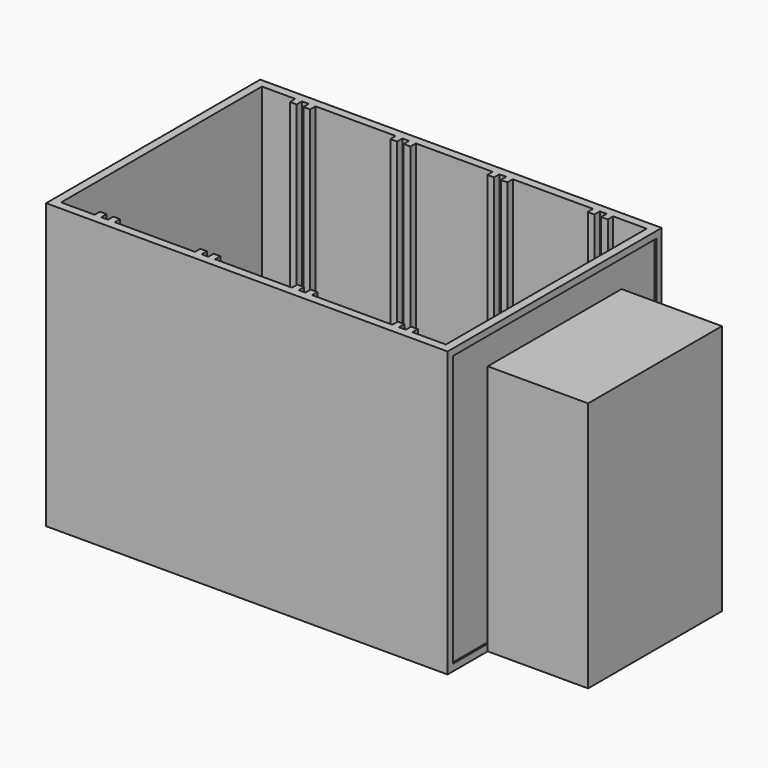
from build123d import *

# Parameters (mm, degrees)
F0_W           = 120
F0_H           = 80
F1_DEPTH       = 85
F2_T           = -2.5
F3_W           = 2
F3_H           = 2
F4_DEPTH       = 85
F5_W           = 30
F5_H           = 50
F6_DEPTH       = 75
F7_T           = -2
F7_2_T         = 2
F7_2_T3_DEPTH  = 86.5
F7_2_T5_DEPTH  = 14
F7_2_T7_DEPTH  = 6
F7_2_T9_DEPTH  = 28
F7_2_T11_DEPTH = 6
F7_2_T13_DEPTH = 27
F7_2_T15_DEPTH = 6
F7_2_T17_DEPTH = 28
F7_2_T19_DEPTH = 6
F7_2_T21_DEPTH = 14
F7_2_T23_DEPTH = 79
F7_2_T25_DEPTH = 6
F7_2_T27_DEPTH = 6
F7_2_T29_DEPTH = 6
F7_2_T31_DEPTH = 6
F7_2_T33_DEPTH = 6
F7_2_T35_DEPTH = 6
F7_2_T37_DEPTH = 6
F7_2_T39_DEPTH = 6
F7_2_T41_DEPTH = 6
F7_2_T43_DEPTH = 6


# Not quite as in the source:
# - a shell that OpenCascade refuses in one call is made with other operations: the cavity is built on its own and cut out


with BuildPart() as f1:
    # F0 (on Top) → F1 (new body)
    with BuildSketch(Plane.XY):
        Rectangle(F0_W, F0_H)
    extrude(amount=F1_DEPTH)

    # F2
    f2_openings = [f1.faces().sort_by_distance(p)[0] for p in [
        (0, 0, 85),
    ]]
    offset(amount=F2_T, openings=f2_openings)

    # F3 (on Top) → F4 (join)
    with BuildSketch(Plane.XY):
        with Locations((-46.5, -36.5)):
            Rectangle(F3_W, F3_H)
        with Locations((-42.5, -36.5)):
            Rectangle(F3_W, F3_H)
        with Locations((-16.5, -36.5)):
            Rectangle(F3_W, F3_H)
        with Locations((-12.5, -36.5)):
            Rectangle(F3_W, F3_H)
        with Locations((42.5, -36.5)):
            Rectangle(F3_W, F3_H)
        with Locations((46.5, -36.5)):
            Rectangle(F3_W, F3_H)
        with Locations((12.5, -36.5)):
            Rectangle(F3_W, F3_H)
        with Locations((16.5, -36.5)):
            Rectangle(F3_W, F3_H)
        with Locations((-46.5, 36.5)):
            Rectangle(F3_W, F3_H)
        with Locations((42.5, 36.5)):
            Rectangle(F3_W, F3_H)
        with Locations((-16.5, 36.5)):
            Rectangle(F3_W, F3_H)
        with Locations((-42.5, 36.5)):
            Rectangle(F3_W, F3_H)
        with Locations((-12.5, 36.5)):
            Rectangle(F3_W, F3_H)
        with Locations((46.5, 36.5)):
            Rectangle(F3_W, F3_H)
        with Locations((16.5, 36.5)):
            Rectangle(F3_W, F3_H)
        with Locations((12.5, 36.5)):
            Rectangle(F3_W, F3_H)
    extrude(amount=F4_DEPTH)

    # F7#2: shell of thickness 2, made by hand


with BuildPart() as f6:
    # F5 (on Top) → F6 (new body)
    with BuildSketch(Plane.XY):
        with Locations((75, 0)):
            Rectangle(F5_W, F5_H)
    extrude(amount=F6_DEPTH)

    # F7
    f7_openings = [f6.faces().sort_by_distance(p)[0] for p in [
        (60, 0, 37.5),
    ]]
    offset(amount=F7_T, openings=f7_openings)


with BuildPart() as f7_2_core1:
    # F7_2_t2: copy of F1
    add(f1.part)

    # the walls: a layer under each face that stays
    f7_2_faces = [f7_2_core1.faces().sort_by_distance(p)[0] for p in [
        (0, -40, 42.5),
        (-60, 0, 42.5),
        (0, 0, 0),
        (-16, -37.3333333333, 85),
        (0, 40, 42.5),
        (-52.5, -37.5, 43.75),
        (-44.5, -37.5, 43.75),
        (-29.5, -37.5, 43.75),
        (-14.5, -37.5, 43.75),
        (0, -37.5, 43.75),
        (14.5, -37.5, 43.75),
        (29.5, -37.5, 43.75),
        (44.5, -37.5, 43.75),
        (52.5, -37.5, 43.75),
        (-57.5, 0, 43.75),
        (52.5, 37.5, 43.75),
        (44.5, 37.5, 43.75),
        (29.5, 37.5, 43.75),
        (14.5, 37.5, 43.75),
        (0, 37.5, 43.75),
        (-14.5, 37.5, 43.75),
        (-29.5, 37.5, 43.75),
        (-44.5, 37.5, 43.75),
        (-52.5, 37.5, 43.75),
        (57.5, 0, 43.75),
        (0, 0, 2.5),
        (-47.5, -36.5, 43.75),
        (-45.5, -36.5, 43.75),
        (-46.5, -35.5, 43.75),
        (-43.5, -36.5, 43.75),
        (-41.5, -36.5, 43.75),
        (-42.5, -35.5, 43.75),
        (-17.5, -36.5, 43.75),
        (-15.5, -36.5, 43.75),
        (-16.5, -35.5, 43.75),
        (-13.5, -36.5, 43.75),
        (-11.5, -36.5, 43.75),
        (-12.5, -35.5, 43.75),
        (11.5, -36.5, 43.75),
        (12.5, -35.5, 43.75),
        (13.5, -36.5, 43.75),
        (15.5, -36.5, 43.75),
        (17.5, -36.5, 43.75),
        (16.5, -35.5, 43.75),
        (41.5, -36.5, 43.75),
        (43.5, -36.5, 43.75),
        (42.5, -35.5, 43.75),
        (45.5, -36.5, 43.75),
        (47.5, -36.5, 43.75),
        (46.5, -35.5, 43.75),
        (47.5, 36.5, 43.75),
        (46.5, 35.5, 43.75),
        (45.5, 36.5, 43.75),
        (43.5, 36.5, 43.75),
        (42.5, 35.5, 43.75),
        (41.5, 36.5, 43.75),
        (17.5, 36.5, 43.75),
        (15.5, 36.5, 43.75),
        (16.5, 35.5, 43.75),
        (13.5, 36.5, 43.75),
        (11.5, 36.5, 43.75),
        (12.5, 35.5, 43.75),
        (-11.5, 36.5, 43.75),
        (-13.5, 36.5, 43.75),
        (-12.5, 35.5, 43.75),
        (-15.5, 36.5, 43.75),
        (-17.5, 36.5, 43.75),
        (-16.5, 35.5, 43.75),
        (-41.5, 36.5, 43.75),
        (-43.5, 36.5, 43.75),
        (-42.5, 35.5, 43.75),
        (-45.5, 36.5, 43.75),
        (-46.5, 35.5, 43.75),
        (-47.5, 36.5, 43.75),
    ]]
    thicken(f7_2_faces, amount=-F7_2_T, mode=Mode.SUBTRACT)

    # F7_2_s4 → F7_2_t3 (cut)
    with BuildSketch(Plane.XY.offset(0.5)):
        Polygon((-57.48, -37.48), (-57.5, -39.5), (-59.5, -39.5), (-59.5, -37.5), align=None)
        Polygon((-47.52, -37.48), (-47.5, -39.5), (-45.5, -39.5), (-45.5, -37.5), align=None)
        Polygon((-45.48, -37.48), (-45.5, -39.5), (-47.5, -39.5), (-47.5, -37.5), align=None)
        Polygon((-43.52, -37.48), (-43.5, -39.5), (-41.5, -39.5), (-41.5, -37.5), align=None)
        Polygon((-41.48, -37.48), (-41.5, -39.5), (-43.5, -39.5), (-43.5, -37.5), align=None)
        Polygon((-17.52, -37.48), (-17.5, -39.5), (-15.5, -39.5), (-15.5, -37.5), align=None)
        Polygon((-15.48, -37.48), (-15.5, -39.5), (-17.5, -39.5), (-17.5, -37.5), align=None)
        Polygon((-13.52, -37.48), (-13.5, -39.5), (-11.5, -39.5), (-11.5, -37.5), align=None)
        Polygon((-11.48, -37.48), (-11.5, -39.5), (-13.5, -39.5), (-13.5, -37.5), align=None)
        Polygon((11.48, -37.48), (11.5, -39.5), (13.5, -39.5), (13.5, -37.5), align=None)
        Polygon((13.52, -37.48), (13.5, -39.5), (11.5, -39.5), (11.5, -37.5), align=None)
        Polygon((15.48, -37.48), (15.5, -39.5), (17.5, -39.5), (17.5, -37.5), align=None)
        Polygon((17.52, -37.48), (17.5, -39.5), (15.5, -39.5), (15.5, -37.5), align=None)
        Polygon((41.48, -37.48), (41.5, -39.5), (43.5, -39.5), (43.5, -37.5), align=None)
        Polygon((43.52, -37.48), (43.5, -39.5), (41.5, -39.5), (41.5, -37.5), align=None)
        Polygon((45.48, -37.48), (45.5, -39.5), (47.5, -39.5), (47.5, -37.5), align=None)
        Polygon((47.52, -37.48), (47.5, -39.5), (45.5, -39.5), (45.5, -37.5), align=None)
        Polygon((57.48, -37.48), (57.5, -39.5), (59.5, -39.5), (59.5, -37.5), align=None)
        Polygon((-57.48, 37.48), (-59.5, 37.5), (-59.5, 39.5), (-57.5, 39.5), align=None)
        Polygon((57.48, 37.48), (57.5, 39.5), (59.5, 39.5), (59.5, 37.5), align=None)
        Polygon((47.52, 37.48), (47.5, 39.5), (45.5, 39.5), (45.5, 37.5), align=None)
        Polygon((45.48, 37.48), (45.5, 39.5), (47.5, 39.5), (47.5, 37.5), align=None)
        Polygon((43.52, 37.48), (43.5, 39.5), (41.5, 39.5), (41.5, 37.5), align=None)
        Polygon((41.48, 37.48), (41.5, 39.5), (43.5, 39.5), (43.5, 37.5), align=None)
        Polygon((17.52, 37.48), (17.5, 39.5), (15.5, 39.5), (15.5, 37.5), align=None)
        Polygon((15.48, 37.48), (15.5, 39.5), (17.5, 39.5), (17.5, 37.5), align=None)
        Polygon((13.52, 37.48), (13.5, 39.5), (11.5, 39.5), (11.5, 37.5), align=None)
        Polygon((11.48, 37.48), (11.5, 39.5), (13.5, 39.5), (13.5, 37.5), align=None)
        Polygon((-11.48, 37.48), (-11.5, 39.5), (-13.5, 39.5), (-13.5, 37.5), align=None)
        Polygon((-13.52, 37.48), (-13.5, 39.5), (-11.5, 39.5), (-11.5, 37.5), align=None)
        Polygon((-15.48, 37.48), (-15.5, 39.5), (-17.5, 39.5), (-17.5, 37.5), align=None)
        Polygon((-17.52, 37.48), (-17.5, 39.5), (-15.5, 39.5), (-15.5, 37.5), align=None)
        Polygon((-41.48, 37.48), (-41.5, 39.5), (-43.5, 39.5), (-43.5, 37.5), align=None)
        Polygon((-43.52, 37.48), (-43.5, 39.5), (-41.5, 39.5), (-41.5, 37.5), align=None)
        Polygon((-45.48, 37.48), (-45.5, 39.5), (-47.5, 39.5), (-47.5, 37.5), align=None)
        Polygon((-47.52, 37.48), (-47.5, 39.5), (-45.5, 39.5), (-45.5, 37.5), align=None)
    extrude(amount=F7_2_T3_DEPTH, mode=Mode.SUBTRACT)

    # F7_2_s6 → F7_2_t5 (cut)
    with BuildSketch(Plane.YZ.offset(-59.5)):
        Polygon((-37.48, 2.52), (-39.5, 2.5), (-39.5, 0.5), (-37.5, 0.5), align=None)
        Polygon((37.48, 2.52), (39.5, 2.5), (39.5, 0.5), (37.5, 0.5), align=None)
    extrude(amount=F7_2_T5_DEPTH, mode=Mode.SUBTRACT)

    # F7_2_s8 → F7_2_t7 (cut)
    with BuildSketch(Plane.YZ.offset(-47.5)):
        Polygon((-37.48, 2.52), (-39.5, 2.5), (-39.5, 0.5), (-37.5, 0.5), align=None)
        Polygon((37.48, 2.52), (39.5, 2.5), (39.5, 0.5), (37.5, 0.5), align=None)
    extrude(amount=F7_2_T7_DEPTH, mode=Mode.SUBTRACT)

    # F7_2_s10 → F7_2_t9 (cut)
    with BuildSketch(Plane.YZ.offset(-43.5)):
        Polygon((-37.48, 2.52), (-39.5, 2.5), (-39.5, 0.5), (-37.5, 0.5), align=None)
        Polygon((37.48, 2.52), (39.5, 2.5), (39.5, 0.5), (37.5, 0.5), align=None)
    extrude(amount=F7_2_T9_DEPTH, mode=Mode.SUBTRACT)

    # F7_2_s12 → F7_2_t11 (cut)
    with BuildSketch(Plane.YZ.offset(-17.5)):
        Polygon((-37.48, 2.52), (-39.5, 2.5), (-39.5, 0.5), (-37.5, 0.5), align=None)
        Polygon((37.48, 2.52), (39.5, 2.5), (39.5, 0.5), (37.5, 0.5), align=None)
    extrude(amount=F7_2_T11_DEPTH, mode=Mode.SUBTRACT)

    # F7_2_s14 → F7_2_t13 (cut)
    with BuildSketch(Plane.YZ.offset(-13.5)):
        Polygon((-37.48, 2.52), (-39.5, 2.5), (-39.5, 0.5), (-37.5, 0.5), align=None)
        Polygon((37.48, 2.52), (39.5, 2.5), (39.5, 0.5), (37.5, 0.5), align=None)
    extrude(amount=F7_2_T13_DEPTH, mode=Mode.SUBTRACT)

    # F7_2_s16 → F7_2_t15 (cut)
    with BuildSketch(Plane.YZ.offset(11.5)):
        Polygon((-37.48, 2.52), (-39.5, 2.5), (-39.5, 0.5), (-37.5, 0.5), align=None)
        Polygon((37.48, 2.52), (39.5, 2.5), (39.5, 0.5), (37.5, 0.5), align=None)
    extrude(amount=F7_2_T15_DEPTH, mode=Mode.SUBTRACT)

    # F7_2_s18 → F7_2_t17 (cut)
    with BuildSketch(Plane.YZ.offset(15.5)):
        Polygon((-37.48, 2.52), (-39.5, 2.5), (-39.5, 0.5), (-37.5, 0.5), align=None)
        Polygon((37.48, 2.52), (39.5, 2.5), (39.5, 0.5), (37.5, 0.5), align=None)
    extrude(amount=F7_2_T17_DEPTH, mode=Mode.SUBTRACT)

    # F7_2_s20 → F7_2_t19 (cut)
    with BuildSketch(Plane.YZ.offset(41.5)):
        Polygon((-37.48, 2.52), (-39.5, 2.5), (-39.5, 0.5), (-37.5, 0.5), align=None)
        Polygon((37.48, 2.52), (39.5, 2.5), (39.5, 0.5), (37.5, 0.5), align=None)
    extrude(amount=F7_2_T19_DEPTH, mode=Mode.SUBTRACT)

    # F7_2_s22 → F7_2_t21 (cut)
    with BuildSketch(Plane.YZ.offset(45.5)):
        Polygon((-37.48, 2.52), (-39.5, 2.5), (-39.5, 0.5), (-37.5, 0.5), align=None)
        Polygon((37.48, 2.52), (39.5, 2.5), (39.5, 0.5), (37.5, 0.5), align=None)
    extrude(amount=F7_2_T21_DEPTH, mode=Mode.SUBTRACT)

    # F7_2_s24 → F7_2_t23 (cut)
    with BuildSketch(Plane.XZ.offset(-39.5)):
        Polygon((-57.48, 2.52), (-59.5, 2.5), (-59.5, 0.5), (-57.5, 0.5), align=None)
        Polygon((57.48, 2.52), (59.5, 2.5), (59.5, 0.5), (57.5, 0.5), align=None)
    extrude(amount=F7_2_T23_DEPTH, mode=Mode.SUBTRACT)

    # F7_2_s26 → F7_2_t25 (cut)
    with BuildSketch(Plane.XZ.offset(-39.5)):
        Polygon((-47.52, 2.52), (-47.5, 0.5), (-45.5, 0.5), (-45.5, 2.5), align=None)
        Polygon((-45.48, 2.52), (-45.5, 0.5), (-47.5, 0.5), (-47.5, 2.5), align=None)
        Polygon((-43.52, 2.52), (-43.5, 0.5), (-41.5, 0.5), (-41.5, 2.5), align=None)
        Polygon((-41.48, 2.52), (-41.5, 0.5), (-43.5, 0.5), (-43.5, 2.5), align=None)
        Polygon((-17.52, 2.52), (-17.5, 0.5), (-15.5, 0.5), (-15.5, 2.5), align=None)
        Polygon((-15.48, 2.52), (-15.5, 0.5), (-17.5, 0.5), (-17.5, 2.5), align=None)
        Polygon((-13.52, 2.52), (-13.5, 0.5), (-11.5, 0.5), (-11.5, 2.5), align=None)
        Polygon((-11.48, 2.52), (-11.5, 0.5), (-13.5, 0.5), (-13.5, 2.5), align=None)
        Polygon((11.48, 2.52), (11.5, 0.5), (13.5, 0.5), (13.5, 2.5), align=None)
        Polygon((13.52, 2.52), (13.5, 0.5), (11.5, 0.5), (11.5, 2.5), align=None)
        Polygon((15.48, 2.52), (15.5, 0.5), (17.5, 0.5), (17.5, 2.5), align=None)
        Polygon((17.52, 2.52), (17.5, 0.5), (15.5, 0.5), (15.5, 2.5), align=None)
        Polygon((41.48, 2.52), (41.5, 0.5), (43.5, 0.5), (43.5, 2.5), align=None)
        Polygon((43.52, 2.52), (43.5, 0.5), (41.5, 0.5), (41.5, 2.5), align=None)
        Polygon((45.48, 2.52), (45.5, 0.5), (47.5, 0.5), (47.5, 2.5), align=None)
        Polygon((47.52, 2.52), (47.5, 0.5), (45.5, 0.5), (45.5, 2.5), align=None)
    extrude(amount=F7_2_T25_DEPTH, mode=Mode.SUBTRACT)

    # F7_2_s28 → F7_2_t27 (cut)
    with BuildSketch(Plane.YZ.offset(-49.5)):
        Polygon((35.48, 2.52), (35.5, 0.5), (37.5, 0.5), (37.5, 2.5), align=None)
        Polygon((-35.48, 2.52), (-35.5, 0.5), (-37.5, 0.5), (-37.5, 2.5), align=None)
    extrude(amount=F7_2_T27_DEPTH, mode=Mode.SUBTRACT)

    # F7_2_s30 → F7_2_t29 (cut)
    with BuildSketch(Plane.YZ.offset(-45.5)):
        Polygon((35.48, 2.52), (35.5, 0.5), (37.5, 0.5), (37.5, 2.5), align=None)
        Polygon((-35.48, 2.52), (-35.5, 0.5), (-37.5, 0.5), (-37.5, 2.5), align=None)
    extrude(amount=F7_2_T29_DEPTH, mode=Mode.SUBTRACT)

    # F7_2_s32 → F7_2_t31 (cut)
    with BuildSketch(Plane.YZ.offset(-19.5)):
        Polygon((35.48, 2.52), (35.5, 0.5), (37.5, 0.5), (37.5, 2.5), align=None)
        Polygon((-35.48, 2.52), (-35.5, 0.5), (-37.5, 0.5), (-37.5, 2.5), align=None)
    extrude(amount=F7_2_T31_DEPTH, mode=Mode.SUBTRACT)

    # F7_2_s34 → F7_2_t33 (cut)
    with BuildSketch(Plane.YZ.offset(-15.5)):
        Polygon((35.48, 2.52), (35.5, 0.5), (37.5, 0.5), (37.5, 2.5), align=None)
        Polygon((-35.48, 2.52), (-35.5, 0.5), (-37.5, 0.5), (-37.5, 2.5), align=None)
    extrude(amount=F7_2_T33_DEPTH, mode=Mode.SUBTRACT)

    # F7_2_s36 → F7_2_t35 (cut)
    with BuildSketch(Plane.YZ.offset(9.5)):
        Polygon((35.48, 2.52), (35.5, 0.5), (37.5, 0.5), (37.5, 2.5), align=None)
        Polygon((-35.48, 2.52), (-35.5, 0.5), (-37.5, 0.5), (-37.5, 2.5), align=None)
    extrude(amount=F7_2_T35_DEPTH, mode=Mode.SUBTRACT)

    # F7_2_s38 → F7_2_t37 (cut)
    with BuildSketch(Plane.YZ.offset(13.5)):
        Polygon((35.48, 2.52), (35.5, 0.5), (37.5, 0.5), (37.5, 2.5), align=None)
        Polygon((-35.48, 2.52), (-35.5, 0.5), (-37.5, 0.5), (-37.5, 2.5), align=None)
    extrude(amount=F7_2_T37_DEPTH, mode=Mode.SUBTRACT)

    # F7_2_s40 → F7_2_t39 (cut)
    with BuildSketch(Plane.YZ.offset(39.5)):
        Polygon((35.48, 2.52), (35.5, 0.5), (37.5, 0.5), (37.5, 2.5), align=None)
        Polygon((-35.48, 2.52), (-35.5, 0.5), (-37.5, 0.5), (-37.5, 2.5), align=None)
    extrude(amount=F7_2_T39_DEPTH, mode=Mode.SUBTRACT)

    # F7_2_s42 → F7_2_t41 (cut)
    with BuildSketch(Plane.YZ.offset(43.5)):
        Polygon((35.48, 2.52), (35.5, 0.5), (37.5, 0.5), (37.5, 2.5), align=None)
        Polygon((-35.48, 2.52), (-35.5, 0.5), (-37.5, 0.5), (-37.5, 2.5), align=None)
    extrude(amount=F7_2_T41_DEPTH, mode=Mode.SUBTRACT)

    # F7_2_s44 → F7_2_t43 (cut)
    with BuildSketch(Plane.XZ.offset(33.5)):
        Polygon((47.52, 2.52), (47.5, 0.5), (45.5, 0.5), (45.5, 2.5), align=None)
        Polygon((45.48, 2.52), (45.5, 0.5), (47.5, 0.5), (47.5, 2.5), align=None)
        Polygon((43.52, 2.52), (43.5, 0.5), (41.5, 0.5), (41.5, 2.5), align=None)
        Polygon((41.48, 2.52), (41.5, 0.5), (43.5, 0.5), (43.5, 2.5), align=None)
        Polygon((17.52, 2.52), (17.5, 0.5), (15.5, 0.5), (15.5, 2.5), align=None)
        Polygon((15.48, 2.52), (15.5, 0.5), (17.5, 0.5), (17.5, 2.5), align=None)
        Polygon((13.52, 2.52), (13.5, 0.5), (11.5, 0.5), (11.5, 2.5), align=None)
        Polygon((11.48, 2.52), (11.5, 0.5), (13.5, 0.5), (13.5, 2.5), align=None)
        Polygon((-11.48, 2.52), (-11.5, 0.5), (-13.5, 0.5), (-13.5, 2.5), align=None)
        Polygon((-13.52, 2.52), (-13.5, 0.5), (-11.5, 0.5), (-11.5, 2.5), align=None)
        Polygon((-15.48, 2.52), (-15.5, 0.5), (-17.5, 0.5), (-17.5, 2.5), align=None)
        Polygon((-17.52, 2.52), (-17.5, 0.5), (-15.5, 0.5), (-15.5, 2.5), align=None)
        Polygon((-41.48, 2.52), (-41.5, 0.5), (-43.5, 0.5), (-43.5, 2.5), align=None)
        Polygon((-43.52, 2.52), (-43.5, 0.5), (-41.5, 0.5), (-41.5, 2.5), align=None)
        Polygon((-45.48, 2.52), (-45.5, 0.5), (-47.5, 0.5), (-47.5, 2.5), align=None)
        Polygon((-47.52, 2.52), (-47.5, 0.5), (-45.5, 0.5), (-45.5, 2.5), align=None)
    extrude(amount=F7_2_T43_DEPTH, mode=Mode.SUBTRACT)


with BuildPart() as f1_1:
    add(f1.part)

    # what is left inside the walls is the cavity
    f7_2_cavity = [f7_2_core1.part.solids().sort_by_distance(p)[0] for p in [
        (59.98, 0, 56),
    ]]
    add(f7_2_cavity, mode=Mode.SUBTRACT)


solid = Compound([f6.part, f1_1.part])
